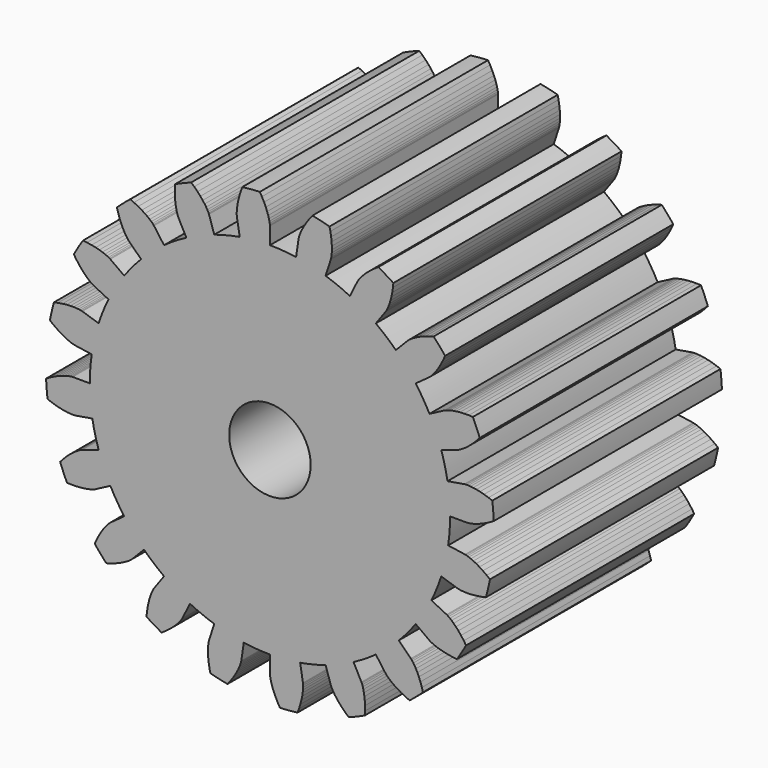
from build123d import *

# Parameters (mm, degrees)
F0_R     = 5
F1_DEPTH = 35


# Not quite as in the source:
# - ends of sketch curves that miss each other by under 0.0002 mm in the source are joined


with BuildPart() as f1:
    # F0 (on Front) → F1 (new body)
    with BuildSketch(Plane.XZ):
        with BuildLine():
            Line((-22.108, 0), (-24.2, 0))
            Line((-24.2, 0), (-24.23024, -0.00108))
            Line((-24.23024, -0.00108), (-24.32068, -0.00824))
            Line((-24.32068, -0.00824), (-24.47072, -0.02744))
            Line((-24.47072, -0.02744), (-24.67916, -0.06464))
            Line((-24.67916, -0.06464), (-24.94448, -0.12572))
            Line((-24.94448, -0.12572), (-25.2646, -0.2164))
            Line((-25.2646, -0.2164), (-25.63716, -0.34232))
            Line((-25.63716, -0.34232), (-26.05924, -0.50884))
            Line((-26.05924, -0.50884), (-26.52756, -0.72116))
            Line((-26.52756, -0.72116), (-27.03852, -0.98436))
            Line((-27.03852, -0.98436), (-27.4722, -1.23588))
            ThreePointArc((-27.4722, -1.23588), (-27.4025906987, -2.3125792959), (-27.2907844004, -3.3857180647))
            Line((-27.2907844004, -3.3857180647), (-26.82104, -3.561))
            Line((-26.82104, -3.561), (-26.27324, -3.73484))
            Line((-26.27324, -3.73484), (-25.77592, -3.86568))
            Line((-25.77592, -3.86568), (-25.33192, -3.95912))
            Line((-25.33192, -3.95912), (-24.94356, -4.0208))
            Line((-24.94356, -4.0208), (-24.61272, -4.05656))
            Line((-24.61272, -4.05656), (-24.34096, -4.07228))
            Line((-24.34096, -4.07228), (-24.1292, -4.07404))
            Line((-24.1292, -4.07404), (-23.97808, -4.06784))
            Line((-23.97808, -4.06784), (-23.88772, -4.05972))
            Line((-23.88772, -4.05972), (-23.85772, -4.05572))
            Line((-23.85772, -4.05572), (-21.79532, -3.70512))
            ThreePointArc((-21.79532, -3.70512), (-21.4676323683, -5.2824638663), (-21.0259540931, -6.8317580807))
            Line((-21.0259540931, -6.8317580807), (-23.01556, -7.4782))
            Line((-23.01556, -7.4782), (-23.044, -7.4886))
            Line((-23.044, -7.4886), (-23.1278, -7.52336))
            Line((-23.1278, -7.52336), (-23.26456, -7.58796))
            Line((-23.26456, -7.58796), (-23.45132, -7.68776))
            Line((-23.45132, -7.68776), (-23.68476, -7.82784))
            Line((-23.68476, -7.82784), (-23.9612, -8.013))
            Line((-23.9612, -8.013), (-24.2766, -8.24788))
            Line((-24.2766, -8.24788), (-24.62656, -8.53668))
            Line((-24.62656, -8.53668), (-25.00636, -8.88336))
            Line((-25.00636, -8.88336), (-25.41096, -9.29152))
            Line((-25.41096, -9.29152), (-25.74572, -9.6648))
            ThreePointArc((-25.74572, -9.6648), (-25.3467827469, -10.6672678967), (-24.9088370823, -11.653318635))
            Line((-24.9088370823, -11.653318635), (-24.40792, -11.67488))
            Line((-24.40792, -11.67488), (-23.8332, -11.67092))
            Line((-23.8332, -11.67092), (-23.3198, -11.64168))
            Line((-23.3198, -11.64168), (-22.86864, -11.59332))
            Line((-22.86864, -11.59332), (-22.48024, -11.532))
            Line((-22.48024, -11.532), (-22.15456, -11.46376))
            Line((-22.15456, -11.46376), (-21.8912, -11.39476))
            Line((-21.8912, -11.39476), (-21.68932, -11.331))
            Line((-21.68932, -11.331), (-21.54752, -11.27836))
            Line((-21.54752, -11.27836), (-21.46404, -11.24272))
            Line((-21.46404, -11.24272), (-21.43676, -11.22964))
            Line((-21.43676, -11.22964), (-19.58364, -10.25888))
            ThreePointArc((-19.58364, -10.25888), (-18.7845703543, -11.6577691093), (-17.8857502251, -12.9947528981))
            Line((-17.8857502251, -12.9947528981), (-19.5782, -14.2244))
            Line((-19.5782, -14.2244), (-19.60204, -14.24308))
            Line((-19.60204, -14.24308), (-19.671, -14.302))
            Line((-19.671, -14.302), (-19.78112, -14.40572))
            Line((-19.78112, -14.40572), (-19.92788, -14.55836))
            Line((-19.92788, -14.55836), (-20.1066, -14.76368))
            Line((-20.1066, -14.76368), (-20.31232, -15.02524))
            Line((-20.31232, -15.02524), (-20.53968, -15.34608))
            Line((-20.53968, -15.34608), (-20.78328, -15.72888))
            Line((-20.78328, -15.72888), (-21.03736, -16.17596))
            Line((-21.03736, -16.17596), (-21.29604, -16.6892))
            Line((-21.29604, -16.6892), (-21.49904, -17.1476))
            ThreePointArc((-21.49904, -17.1476), (-20.8098683635, -17.9777467635), (-20.0886483796, -18.7802078338))
            Line((-20.0886483796, -18.7802078338), (-19.6056, -18.64592))
            Line((-19.6056, -18.64592), (-19.06024, -18.46456))
            Line((-19.06024, -18.46456), (-18.58096, -18.27812))
            Line((-18.58096, -18.27812), (-18.16684, -18.09272))
            Line((-18.16684, -18.09272), (-17.8164, -17.91436))
            Line((-17.8164, -17.91436), (-17.52776, -17.74884))
            Line((-17.52776, -17.74884), (-17.2986, -17.6018))
            Line((-17.2986, -17.6018), (-17.12628, -17.47876))
            Line((-17.12628, -17.47876), (-17.00768, -17.38492))
            Line((-17.00768, -17.38492), (-16.93932, -17.3252))
            Line((-16.93932, -17.3252), (-16.9174, -17.30436))
            Line((-16.9174, -17.30436), (-15.45496, -15.80848))
            ThreePointArc((-15.45496, -15.80848), (-14.2627230801, -16.8919624183), (-12.9947528981, -17.8857502251))
            Line((-12.9947528981, -17.8857502251), (-14.2244, -19.5782))
            Line((-14.2244, -19.5782), (-14.24128, -19.60332))
            Line((-14.24128, -19.60332), (-14.28868, -19.68068))
            Line((-14.28868, -19.68068), (-14.36132, -19.81336))
            Line((-14.36132, -19.81336), (-14.45376, -20.00388))
            Line((-14.45376, -20.00388), (-14.56028, -20.2544))
            Line((-14.56028, -20.2544), (-14.67508, -20.56672))
            Line((-14.67508, -20.56672), (-14.7922, -20.94208))
            Line((-14.7922, -20.94208), (-14.9056, -21.38144))
            Line((-14.9056, -21.38144), (-15.00908, -21.88516))
            Line((-15.00908, -21.88516), (-15.09648, -22.4532))
            Line((-15.09648, -22.4532), (-15.14792, -22.95192))
            ThreePointArc((-15.14792, -22.95192), (-14.2359384688, -23.5284520509), (-13.3020446076, -24.068768337))
            Line((-13.3020446076, -24.068768337), (-12.88412, -23.7918))
            Line((-12.88412, -23.7918), (-12.42148, -23.45076))
            Line((-12.42148, -23.45076), (-12.02332, -23.12536))
            Line((-12.02332, -23.12536), (-11.68676, -22.82108))
            Line((-11.68676, -22.82108), (-11.40856, -22.54312))
            Line((-11.40856, -22.54312), (-11.1852, -22.29652))
            Line((-11.1852, -22.29652), (-11.01268, -22.08588))
            Line((-11.01268, -22.08588), (-10.88684, -21.9156))
            Line((-10.88684, -21.9156), (-10.80304, -21.78968))
            Line((-10.80304, -21.78968), (-10.75648, -21.7118))
            Line((-10.75648, -21.7118), (-10.74208, -21.6852))
            Line((-10.74208, -21.6852), (-9.81348, -19.8106))
            ThreePointArc((-9.81348, -19.8106), (-8.3447718051, -20.472626786), (-6.8317580807, -21.0259540931))
            Line((-6.8317580807, -21.0259540931), (-7.4782, -23.01556))
            Line((-7.4782, -23.01556), (-7.48652, -23.04464))
            Line((-7.48652, -23.04464), (-7.50768, -23.13292))
            Line((-7.50768, -23.13292), (-7.53576, -23.28152))
            Line((-7.53576, -23.28152), (-7.5648, -23.49124))
            Line((-7.5648, -23.49124), (-7.58872, -23.76244))
            Line((-7.58872, -23.76244), (-7.6014, -24.09496))
            Line((-7.6014, -24.09496), (-7.59676, -24.48816))
            Line((-7.59676, -24.48816), (-7.56884, -24.94104))
            Line((-7.56884, -24.94104), (-7.5116, -25.45208))
            Line((-7.5116, -25.45208), (-7.4192, -26.01932))
            Line((-7.4192, -26.01932), (-7.314, -26.50952))
            ThreePointArc((-7.314, -26.50952), (-6.2684865248, -26.7760354924), (-5.2133200442, -27.0013202291))
            Line((-5.2133200442, -27.0013202291), (-4.90144, -26.60876))
            Line((-4.90144, -26.60876), (-4.56684, -26.14148))
            Line((-4.56684, -26.14148), (-4.28872, -25.70892))
            Line((-4.28872, -25.70892), (-4.06264, -25.31552))
            Line((-4.06264, -25.31552), (-3.88396, -24.96524))
            Line((-3.88396, -24.96524), (-3.74776, -24.66164))
            Line((-3.74776, -24.66164), (-3.6488, -24.40804))
            Line((-3.6488, -24.40804), (-3.58168, -24.2072))
            Line((-3.58168, -24.2072), (-3.54092, -24.06156))
            Line((-3.54092, -24.06156), (-3.52072, -23.97308))
            Line((-3.52072, -23.97308), (-3.51524, -23.94332))
            Line((-3.51524, -23.94332), (-3.21136, -21.87352))
            ThreePointArc((-3.21136, -21.87352), (-1.6099544582, -22.0493018176), (0, -22.108))
            Line((0, -22.108), (0, -24.2))
            Line((0, -24.2), (0.00108, -24.23024))
            Line((0.00108, -24.23024), (0.00824, -24.32068))
            Line((0.00824, -24.32068), (0.02744, -24.47072))
            Line((0.02744, -24.47072), (0.06464, -24.67916))
            Line((0.06464, -24.67916), (0.12572, -24.94448))
            Line((0.12572, -24.94448), (0.2164, -25.2646))
            Line((0.2164, -25.2646), (0.34232, -25.63716))
            Line((0.34232, -25.63716), (0.50884, -26.05924))
            Line((0.50884, -26.05924), (0.72116, -26.52756))
            Line((0.72116, -26.52756), (0.98436, -27.03852))
            Line((0.98436, -27.03852), (1.23588, -27.4722))
            ThreePointArc((1.23588, -27.4722), (2.3125792959, -27.4025906987), (3.3857180647, -27.2907844004))
            Line((3.3857180647, -27.2907844004), (3.561, -26.82104))
            Line((3.561, -26.82104), (3.73484, -26.27324))
            Line((3.73484, -26.27324), (3.86568, -25.77592))
            Line((3.86568, -25.77592), (3.95912, -25.33192))
            Line((3.95912, -25.33192), (4.0208, -24.94356))
            Line((4.0208, -24.94356), (4.05656, -24.61272))
            Line((4.05656, -24.61272), (4.07228, -24.34096))
            Line((4.07228, -24.34096), (4.07404, -24.1292))
            Line((4.07404, -24.1292), (4.06784, -23.97808))
            Line((4.06784, -23.97808), (4.05972, -23.88772))
            Line((4.05972, -23.88772), (4.05572, -23.85772))
            Line((4.05572, -23.85772), (3.70512, -21.79532))
            ThreePointArc((3.70512, -21.79532), (5.2824638663, -21.4676323683), (6.8317580807, -21.0259540931))
            Line((6.8317580807, -21.0259540931), (7.4782, -23.01556))
            Line((7.4782, -23.01556), (7.4886, -23.044))
            Line((7.4886, -23.044), (7.52336, -23.1278))
            Line((7.52336, -23.1278), (7.58796, -23.26456))
            Line((7.58796, -23.26456), (7.68776, -23.45132))
            Line((7.68776, -23.45132), (7.82784, -23.68476))
            Line((7.82784, -23.68476), (8.013, -23.9612))
            Line((8.013, -23.9612), (8.24788, -24.2766))
            Line((8.24788, -24.2766), (8.53668, -24.62656))
            Line((8.53668, -24.62656), (8.88336, -25.00636))
            Line((8.88336, -25.00636), (9.29152, -25.41096))
            Line((9.29152, -25.41096), (9.6648, -25.74572))
            ThreePointArc((9.6648, -25.74572), (10.6672678967, -25.3467827469), (11.653318635, -24.9088370823))
            Line((11.653318635, -24.9088370823), (11.67488, -24.40792))
            Line((11.67488, -24.40792), (11.67092, -23.8332))
            Line((11.67092, -23.8332), (11.64168, -23.3198))
            Line((11.64168, -23.3198), (11.59332, -22.86864))
            Line((11.59332, -22.86864), (11.532, -22.48024))
            Line((11.532, -22.48024), (11.46376, -22.15456))
            Line((11.46376, -22.15456), (11.39476, -21.8912))
            Line((11.39476, -21.8912), (11.331, -21.68932))
            Line((11.331, -21.68932), (11.27836, -21.54752))
            Line((11.27836, -21.54752), (11.24272, -21.46404))
            Line((11.24272, -21.46404), (11.22964, -21.43676))
            Line((11.22964, -21.43676), (10.25888, -19.58364))
            ThreePointArc((10.25888, -19.58364), (11.6577691093, -18.7845703543), (12.9947528981, -17.8857502251))
            Line((12.9947528981, -17.8857502251), (14.2244, -19.5782))
            Line((14.2244, -19.5782), (14.24308, -19.60204))
            Line((14.24308, -19.60204), (14.302, -19.671))
            Line((14.302, -19.671), (14.40572, -19.78112))
            Line((14.40572, -19.78112), (14.55836, -19.92788))
            Line((14.55836, -19.92788), (14.76368, -20.1066))
            Line((14.76368, -20.1066), (15.02524, -20.31232))
            Line((15.02524, -20.31232), (15.34608, -20.53968))
            Line((15.34608, -20.53968), (15.72888, -20.78328))
            Line((15.72888, -20.78328), (16.17596, -21.03736))
            Line((16.17596, -21.03736), (16.6892, -21.29604))
            Line((16.6892, -21.29604), (17.1476, -21.49904))
            ThreePointArc((17.1476, -21.49904), (17.9777467635, -20.8098683635), (18.7802078338, -20.0886483796))
            Line((18.7802078338, -20.0886483796), (18.64592, -19.6056))
            Line((18.64592, -19.6056), (18.46456, -19.06024))
            Line((18.46456, -19.06024), (18.27812, -18.58096))
            Line((18.27812, -18.58096), (18.09272, -18.16684))
            Line((18.09272, -18.16684), (17.91436, -17.8164))
            Line((17.91436, -17.8164), (17.74884, -17.52776))
            Line((17.74884, -17.52776), (17.6018, -17.2986))
            Line((17.6018, -17.2986), (17.47876, -17.12628))
            Line((17.47876, -17.12628), (17.38492, -17.00768))
            Line((17.38492, -17.00768), (17.3252, -16.93932))
            Line((17.3252, -16.93932), (17.30436, -16.9174))
            Line((17.30436, -16.9174), (15.80848, -15.45496))
            ThreePointArc((15.80848, -15.45496), (16.8919624183, -14.2627230801), (17.8857502251, -12.9947528981))
            Line((17.8857502251, -12.9947528981), (19.5782, -14.2244))
            Line((19.5782, -14.2244), (19.60332, -14.24128))
            Line((19.60332, -14.24128), (19.68068, -14.28868))
            Line((19.68068, -14.28868), (19.81336, -14.36132))
            Line((19.81336, -14.36132), (20.00388, -14.45376))
            Line((20.00388, -14.45376), (20.2544, -14.56028))
            Line((20.2544, -14.56028), (20.56672, -14.67508))
            Line((20.56672, -14.67508), (20.94208, -14.7922))
            Line((20.94208, -14.7922), (21.38144, -14.9056))
            Line((21.38144, -14.9056), (21.88516, -15.00908))
            Line((21.88516, -15.00908), (22.4532, -15.09648))
            Line((22.4532, -15.09648), (22.95192, -15.14792))
            ThreePointArc((22.95192, -15.14792), (23.5284520509, -14.2359384688), (24.068768337, -13.3020446076))
            Line((24.068768337, -13.3020446076), (23.7918, -12.88412))
            Line((23.7918, -12.88412), (23.45076, -12.42148))
            Line((23.45076, -12.42148), (23.12536, -12.02332))
            Line((23.12536, -12.02332), (22.82108, -11.68676))
            Line((22.82108, -11.68676), (22.54312, -11.40856))
            Line((22.54312, -11.40856), (22.29652, -11.1852))
            Line((22.29652, -11.1852), (22.08588, -11.01268))
            Line((22.08588, -11.01268), (21.9156, -10.88684))
            Line((21.9156, -10.88684), (21.78968, -10.80304))
            Line((21.78968, -10.80304), (21.7118, -10.75648))
            Line((21.7118, -10.75648), (21.6852, -10.74208))
            Line((21.6852, -10.74208), (19.8106, -9.81348))
            ThreePointArc((19.8106, -9.81348), (20.472626786, -8.3447718051), (21.0259540931, -6.8317580807))
            Line((21.0259540931, -6.8317580807), (23.01556, -7.4782))
            Line((23.01556, -7.4782), (23.04464, -7.48652))
            Line((23.04464, -7.48652), (23.13292, -7.50768))
            Line((23.13292, -7.50768), (23.28152, -7.53576))
            Line((23.28152, -7.53576), (23.49124, -7.5648))
            Line((23.49124, -7.5648), (23.76244, -7.58872))
            Line((23.76244, -7.58872), (24.09496, -7.6014))
            Line((24.09496, -7.6014), (24.48816, -7.59676))
            Line((24.48816, -7.59676), (24.94104, -7.56884))
            Line((24.94104, -7.56884), (25.45208, -7.5116))
            Line((25.45208, -7.5116), (26.01932, -7.4192))
            Line((26.01932, -7.4192), (26.50952, -7.314))
            ThreePointArc((26.50952, -7.314), (26.7760354924, -6.2684865248), (27.0013202291, -5.2133200442))
            Line((27.0013202291, -5.2133200442), (26.60876, -4.90144))
            Line((26.60876, -4.90144), (26.14148, -4.56684))
            Line((26.14148, -4.56684), (25.70892, -4.28872))
            Line((25.70892, -4.28872), (25.31552, -4.06264))
            Line((25.31552, -4.06264), (24.96524, -3.88396))
            Line((24.96524, -3.88396), (24.66164, -3.74776))
            Line((24.66164, -3.74776), (24.40804, -3.6488))
            Line((24.40804, -3.6488), (24.2072, -3.58168))
            Line((24.2072, -3.58168), (24.06156, -3.54092))
            Line((24.06156, -3.54092), (23.97308, -3.52072))
            Line((23.97308, -3.52072), (23.94332, -3.51524))
            Line((23.94332, -3.51524), (21.87352, -3.21136))
            ThreePointArc((21.87352, -3.21136), (22.0493018176, -1.6099544582), (22.108, 0))
            Line((22.108, 0), (24.2, 0))
            Line((24.2, 0), (24.23024, 0.00108))
            Line((24.23024, 0.00108), (24.32068, 0.00824))
            Line((24.32068, 0.00824), (24.47072, 0.02744))
            Line((24.47072, 0.02744), (24.67916, 0.06464))
            Line((24.67916, 0.06464), (24.94448, 0.12572))
            Line((24.94448, 0.12572), (25.2646, 0.2164))
            Line((25.2646, 0.2164), (25.63716, 0.34232))
            Line((25.63716, 0.34232), (26.05924, 0.50884))
            Line((26.05924, 0.50884), (26.52756, 0.72116))
            Line((26.52756, 0.72116), (27.03852, 0.98436))
            Line((27.03852, 0.98436), (27.4722, 1.23588))
            ThreePointArc((27.4722, 1.23588), (27.4025906987, 2.3125792959), (27.2907844004, 3.3857180647))
            Line((27.2907844004, 3.3857180647), (26.82104, 3.561))
            Line((26.82104, 3.561), (26.27324, 3.73484))
            Line((26.27324, 3.73484), (25.77592, 3.86568))
            Line((25.77592, 3.86568), (25.33192, 3.95912))
            Line((25.33192, 3.95912), (24.94356, 4.0208))
            Line((24.94356, 4.0208), (24.61272, 4.05656))
            Line((24.61272, 4.05656), (24.34096, 4.07228))
            Line((24.34096, 4.07228), (24.1292, 4.07404))
            Line((24.1292, 4.07404), (23.97808, 4.06784))
            Line((23.97808, 4.06784), (23.88772, 4.05972))
            Line((23.88772, 4.05972), (23.85772, 4.05572))
            Line((23.85772, 4.05572), (21.79532, 3.70512))
            ThreePointArc((21.79532, 3.70512), (21.4676323683, 5.2824638663), (21.0259540931, 6.8317580807))
            Line((21.0259540931, 6.8317580807), (23.01556, 7.4782))
            Line((23.01556, 7.4782), (23.044, 7.4886))
            Line((23.044, 7.4886), (23.1278, 7.52336))
            Line((23.1278, 7.52336), (23.26456, 7.58796))
            Line((23.26456, 7.58796), (23.45132, 7.68776))
            Line((23.45132, 7.68776), (23.68476, 7.82784))
            Line((23.68476, 7.82784), (23.9612, 8.013))
            Line((23.9612, 8.013), (24.2766, 8.24788))
            Line((24.2766, 8.24788), (24.62656, 8.53668))
            Line((24.62656, 8.53668), (25.00636, 8.88336))
            Line((25.00636, 8.88336), (25.41096, 9.29152))
            Line((25.41096, 9.29152), (25.74572, 9.6648))
            ThreePointArc((25.74572, 9.6648), (25.3467827469, 10.6672678967), (24.9088370823, 11.653318635))
            Line((24.9088370823, 11.653318635), (24.40792, 11.67488))
            Line((24.40792, 11.67488), (23.8332, 11.67092))
            Line((23.8332, 11.67092), (23.3198, 11.64168))
            Line((23.3198, 11.64168), (22.86864, 11.59332))
            Line((22.86864, 11.59332), (22.48024, 11.532))
            Line((22.48024, 11.532), (22.15456, 11.46376))
            Line((22.15456, 11.46376), (21.8912, 11.39476))
            Line((21.8912, 11.39476), (21.68932, 11.331))
            Line((21.68932, 11.331), (21.54752, 11.27836))
            Line((21.54752, 11.27836), (21.46404, 11.24272))
            Line((21.46404, 11.24272), (21.43676, 11.22964))
            Line((21.43676, 11.22964), (19.58364, 10.25888))
            ThreePointArc((19.58364, 10.25888), (18.7845703543, 11.6577691093), (17.8857502251, 12.9947528981))
            Line((17.8857502251, 12.9947528981), (19.5782, 14.2244))
            Line((19.5782, 14.2244), (19.60204, 14.24308))
            Line((19.60204, 14.24308), (19.671, 14.302))
            Line((19.671, 14.302), (19.78112, 14.40572))
            Line((19.78112, 14.40572), (19.92788, 14.55836))
            Line((19.92788, 14.55836), (20.1066, 14.76368))
            Line((20.1066, 14.76368), (20.31232, 15.02524))
            Line((20.31232, 15.02524), (20.53968, 15.34608))
            Line((20.53968, 15.34608), (20.78328, 15.72888))
            Line((20.78328, 15.72888), (21.03736, 16.17596))
            Line((21.03736, 16.17596), (21.29604, 16.6892))
            Line((21.29604, 16.6892), (21.49904, 17.1476))
            ThreePointArc((21.49904, 17.1476), (20.8098683635, 17.9777467635), (20.0886483796, 18.7802078338))
            Line((20.0886483796, 18.7802078338), (19.6056, 18.64592))
            Line((19.6056, 18.64592), (19.06024, 18.46456))
            Line((19.06024, 18.46456), (18.58096, 18.27812))
            Line((18.58096, 18.27812), (18.16684, 18.09272))
            Line((18.16684, 18.09272), (17.8164, 17.91436))
            Line((17.8164, 17.91436), (17.52776, 17.74884))
            Line((17.52776, 17.74884), (17.2986, 17.6018))
            Line((17.2986, 17.6018), (17.12628, 17.47876))
            Line((17.12628, 17.47876), (17.00768, 17.38492))
            Line((17.00768, 17.38492), (16.93932, 17.3252))
            Line((16.93932, 17.3252), (16.9174, 17.30436))
            Line((16.9174, 17.30436), (15.45496, 15.80848))
            ThreePointArc((15.45496, 15.80848), (14.2627230801, 16.8919624183), (12.9947528981, 17.8857502251))
            Line((12.9947528981, 17.8857502251), (14.2244, 19.5782))
            Line((14.2244, 19.5782), (14.24128, 19.60332))
            Line((14.24128, 19.60332), (14.28868, 19.68068))
            Line((14.28868, 19.68068), (14.36132, 19.81336))
            Line((14.36132, 19.81336), (14.45376, 20.00388))
            Line((14.45376, 20.00388), (14.56028, 20.2544))
            Line((14.56028, 20.2544), (14.67508, 20.56672))
            Line((14.67508, 20.56672), (14.7922, 20.94208))
            Line((14.7922, 20.94208), (14.9056, 21.38144))
            Line((14.9056, 21.38144), (15.00908, 21.88516))
            Line((15.00908, 21.88516), (15.09648, 22.4532))
            Line((15.09648, 22.4532), (15.14792, 22.95192))
            ThreePointArc((15.14792, 22.95192), (14.2359384688, 23.5284520509), (13.3020446076, 24.068768337))
            Line((13.3020446076, 24.068768337), (12.88412, 23.7918))
            Line((12.88412, 23.7918), (12.42148, 23.45076))
            Line((12.42148, 23.45076), (12.02332, 23.12536))
            Line((12.02332, 23.12536), (11.68676, 22.82108))
            Line((11.68676, 22.82108), (11.40856, 22.54312))
            Line((11.40856, 22.54312), (11.1852, 22.29652))
            Line((11.1852, 22.29652), (11.01268, 22.08588))
            Line((11.01268, 22.08588), (10.88684, 21.9156))
            Line((10.88684, 21.9156), (10.80304, 21.78968))
            Line((10.80304, 21.78968), (10.75648, 21.7118))
            Line((10.75648, 21.7118), (10.74208, 21.6852))
            Line((10.74208, 21.6852), (9.81348, 19.8106))
            ThreePointArc((9.81348, 19.8106), (8.3447718051, 20.472626786), (6.8317580807, 21.0259540931))
            Line((6.8317580807, 21.0259540931), (7.4782, 23.01556))
            Line((7.4782, 23.01556), (7.48652, 23.04464))
            Line((7.48652, 23.04464), (7.50768, 23.13292))
            Line((7.50768, 23.13292), (7.53576, 23.28152))
            Line((7.53576, 23.28152), (7.5648, 23.49124))
            Line((7.5648, 23.49124), (7.58872, 23.76244))
            Line((7.58872, 23.76244), (7.6014, 24.09496))
            Line((7.6014, 24.09496), (7.59676, 24.48816))
            Line((7.59676, 24.48816), (7.56884, 24.94104))
            Line((7.56884, 24.94104), (7.5116, 25.45208))
            Line((7.5116, 25.45208), (7.4192, 26.01932))
            Line((7.4192, 26.01932), (7.314, 26.50952))
            ThreePointArc((7.314, 26.50952), (6.2684865248, 26.7760354924), (5.2133200442, 27.0013202291))
            Line((5.2133200442, 27.0013202291), (4.90144, 26.60876))
            Line((4.90144, 26.60876), (4.56684, 26.14148))
            Line((4.56684, 26.14148), (4.28872, 25.70892))
            Line((4.28872, 25.70892), (4.06264, 25.31552))
            Line((4.06264, 25.31552), (3.88396, 24.96524))
            Line((3.88396, 24.96524), (3.74776, 24.66164))
            Line((3.74776, 24.66164), (3.6488, 24.40804))
            Line((3.6488, 24.40804), (3.58168, 24.2072))
            Line((3.58168, 24.2072), (3.54092, 24.06156))
            Line((3.54092, 24.06156), (3.52072, 23.97308))
            Line((3.52072, 23.97308), (3.51524, 23.94332))
            Line((3.51524, 23.94332), (3.21136, 21.87352))
            ThreePointArc((3.21136, 21.87352), (1.6099544582, 22.0493018176), (0, 22.108))
            Line((0, 22.108), (0, 24.2))
            Line((0, 24.2), (-0.00108, 24.23024))
            Line((-0.00108, 24.23024), (-0.00824, 24.32068))
            Line((-0.00824, 24.32068), (-0.02744, 24.47072))
            Line((-0.02744, 24.47072), (-0.06464, 24.67916))
            Line((-0.06464, 24.67916), (-0.12572, 24.94448))
            Line((-0.12572, 24.94448), (-0.2164, 25.2646))
            Line((-0.2164, 25.2646), (-0.34232, 25.63716))
            Line((-0.34232, 25.63716), (-0.50884, 26.05924))
            Line((-0.50884, 26.05924), (-0.72116, 26.52756))
            Line((-0.72116, 26.52756), (-0.98436, 27.03852))
            Line((-0.98436, 27.03852), (-1.23588, 27.4722))
            ThreePointArc((-1.23588, 27.4722), (-2.3125792959, 27.4025906987), (-3.3857180647, 27.2907844004))
            Line((-3.3857180647, 27.2907844004), (-3.561, 26.82104))
            Line((-3.561, 26.82104), (-3.73484, 26.27324))
            Line((-3.73484, 26.27324), (-3.86568, 25.77592))
            Line((-3.86568, 25.77592), (-3.95912, 25.33192))
            Line((-3.95912, 25.33192), (-4.0208, 24.94356))
            Line((-4.0208, 24.94356), (-4.05656, 24.61272))
            Line((-4.05656, 24.61272), (-4.07228, 24.34096))
            Line((-4.07228, 24.34096), (-4.07404, 24.1292))
            Line((-4.07404, 24.1292), (-4.06784, 23.97808))
            Line((-4.06784, 23.97808), (-4.05972, 23.88772))
            Line((-4.05972, 23.88772), (-4.05572, 23.85772))
            Line((-4.05572, 23.85772), (-3.70512, 21.79532))
            ThreePointArc((-3.70512, 21.79532), (-5.2824638663, 21.4676323683), (-6.8317580807, 21.0259540931))
            Line((-6.8317580807, 21.0259540931), (-7.4782, 23.01556))
            Line((-7.4782, 23.01556), (-7.4886, 23.044))
            Line((-7.4886, 23.044), (-7.52336, 23.1278))
            Line((-7.52336, 23.1278), (-7.58796, 23.26456))
            Line((-7.58796, 23.26456), (-7.68776, 23.45132))
            Line((-7.68776, 23.45132), (-7.82784, 23.68476))
            Line((-7.82784, 23.68476), (-8.013, 23.9612))
            Line((-8.013, 23.9612), (-8.24788, 24.2766))
            Line((-8.24788, 24.2766), (-8.53668, 24.62656))
            Line((-8.53668, 24.62656), (-8.88336, 25.00636))
            Line((-8.88336, 25.00636), (-9.29152, 25.41096))
            Line((-9.29152, 25.41096), (-9.6648, 25.74572))
            ThreePointArc((-9.6648, 25.74572), (-10.6672678967, 25.3467827469), (-11.653318635, 24.9088370823))
            Line((-11.653318635, 24.9088370823), (-11.67488, 24.40792))
            Line((-11.67488, 24.40792), (-11.67092, 23.8332))
            Line((-11.67092, 23.8332), (-11.64168, 23.3198))
            Line((-11.64168, 23.3198), (-11.59332, 22.86864))
            Line((-11.59332, 22.86864), (-11.532, 22.48024))
            Line((-11.532, 22.48024), (-11.46376, 22.15456))
            Line((-11.46376, 22.15456), (-11.39476, 21.8912))
            Line((-11.39476, 21.8912), (-11.331, 21.68932))
            Line((-11.331, 21.68932), (-11.27836, 21.54752))
            Line((-11.27836, 21.54752), (-11.24272, 21.46404))
            Line((-11.24272, 21.46404), (-11.22964, 21.43676))
            Line((-11.22964, 21.43676), (-10.25888, 19.58364))
            ThreePointArc((-10.25888, 19.58364), (-11.6577691093, 18.7845703543), (-12.9947528981, 17.8857502251))
            Line((-12.9947528981, 17.8857502251), (-14.2244, 19.5782))
            Line((-14.2244, 19.5782), (-14.24308, 19.60204))
            Line((-14.24308, 19.60204), (-14.302, 19.671))
            Line((-14.302, 19.671), (-14.40572, 19.78112))
            Line((-14.40572, 19.78112), (-14.55836, 19.92788))
            Line((-14.55836, 19.92788), (-14.76368, 20.1066))
            Line((-14.76368, 20.1066), (-15.02524, 20.31232))
            Line((-15.02524, 20.31232), (-15.34608, 20.53968))
            Line((-15.34608, 20.53968), (-15.72888, 20.78328))
            Line((-15.72888, 20.78328), (-16.17596, 21.03736))
            Line((-16.17596, 21.03736), (-16.6892, 21.29604))
            Line((-16.6892, 21.29604), (-17.1476, 21.49904))
            ThreePointArc((-17.1476, 21.49904), (-17.9777467635, 20.8098683635), (-18.7802078338, 20.0886483796))
            Line((-18.7802078338, 20.0886483796), (-18.64592, 19.6056))
            Line((-18.64592, 19.6056), (-18.46456, 19.06024))
            Line((-18.46456, 19.06024), (-18.27812, 18.58096))
            Line((-18.27812, 18.58096), (-18.09272, 18.16684))
            Line((-18.09272, 18.16684), (-17.91436, 17.8164))
            Line((-17.91436, 17.8164), (-17.74884, 17.52776))
            Line((-17.74884, 17.52776), (-17.6018, 17.2986))
            Line((-17.6018, 17.2986), (-17.47876, 17.12628))
            Line((-17.47876, 17.12628), (-17.38492, 17.00768))
            Line((-17.38492, 17.00768), (-17.3252, 16.93932))
            Line((-17.3252, 16.93932), (-17.30436, 16.9174))
            Line((-17.30436, 16.9174), (-15.80848, 15.45496))
            ThreePointArc((-15.80848, 15.45496), (-16.8919624183, 14.2627230801), (-17.8857502251, 12.9947528981))
            Line((-17.8857502251, 12.9947528981), (-19.5782, 14.2244))
            Line((-19.5782, 14.2244), (-19.60332, 14.24128))
            Line((-19.60332, 14.24128), (-19.68068, 14.28868))
            Line((-19.68068, 14.28868), (-19.81336, 14.36132))
            Line((-19.81336, 14.36132), (-20.00388, 14.45376))
            Line((-20.00388, 14.45376), (-20.2544, 14.56028))
            Line((-20.2544, 14.56028), (-20.56672, 14.67508))
            Line((-20.56672, 14.67508), (-20.94208, 14.7922))
            Line((-20.94208, 14.7922), (-21.38144, 14.9056))
            Line((-21.38144, 14.9056), (-21.88516, 15.00908))
            Line((-21.88516, 15.00908), (-22.4532, 15.09648))
            Line((-22.4532, 15.09648), (-22.95192, 15.14792))
            ThreePointArc((-22.95192, 15.14792), (-23.5284520509, 14.2359384688), (-24.068768337, 13.3020446076))
            Line((-24.068768337, 13.3020446076), (-23.7918, 12.88412))
            Line((-23.7918, 12.88412), (-23.45076, 12.42148))
            Line((-23.45076, 12.42148), (-23.12536, 12.02332))
            Line((-23.12536, 12.02332), (-22.82108, 11.68676))
            Line((-22.82108, 11.68676), (-22.54312, 11.40856))
            Line((-22.54312, 11.40856), (-22.29652, 11.1852))
            Line((-22.29652, 11.1852), (-22.08588, 11.01268))
            Line((-22.08588, 11.01268), (-21.9156, 10.88684))
            Line((-21.9156, 10.88684), (-21.78968, 10.80304))
            Line((-21.78968, 10.80304), (-21.7118, 10.75648))
            Line((-21.7118, 10.75648), (-21.6852, 10.74208))
            Line((-21.6852, 10.74208), (-19.8106, 9.81348))
            ThreePointArc((-19.8106, 9.81348), (-20.472626786, 8.3447718051), (-21.0259540931, 6.8317580807))
            Line((-21.0259540931, 6.8317580807), (-23.01556, 7.4782))
            Line((-23.01556, 7.4782), (-23.04464, 7.48652))
            Line((-23.04464, 7.48652), (-23.13292, 7.50768))
            Line((-23.13292, 7.50768), (-23.28152, 7.53576))
            Line((-23.28152, 7.53576), (-23.49124, 7.5648))
            Line((-23.49124, 7.5648), (-23.76244, 7.58872))
            Line((-23.76244, 7.58872), (-24.09496, 7.6014))
            Line((-24.09496, 7.6014), (-24.48816, 7.59676))
            Line((-24.48816, 7.59676), (-24.94104, 7.56884))
            Line((-24.94104, 7.56884), (-25.45208, 7.5116))
            Line((-25.45208, 7.5116), (-26.01932, 7.4192))
            Line((-26.01932, 7.4192), (-26.50952, 7.314))
            ThreePointArc((-26.50952, 7.314), (-26.7760354924, 6.2684865248), (-27.0013202291, 5.2133200442))
            Line((-27.0013202291, 5.2133200442), (-26.60876, 4.90144))
            Line((-26.60876, 4.90144), (-26.14148, 4.56684))
            Line((-26.14148, 4.56684), (-25.70892, 4.28872))
            Line((-25.70892, 4.28872), (-25.31552, 4.06264))
            Line((-25.31552, 4.06264), (-24.96524, 3.88396))
            Line((-24.96524, 3.88396), (-24.66164, 3.74776))
            Line((-24.66164, 3.74776), (-24.40804, 3.6488))
            Line((-24.40804, 3.6488), (-24.2072, 3.58168))
            Line((-24.2072, 3.58168), (-24.06156, 3.54092))
            Line((-24.06156, 3.54092), (-23.97308, 3.52072))
            Line((-23.97308, 3.52072), (-23.94332, 3.51524))
            Line((-23.94332, 3.51524), (-21.87352, 3.21136))
            ThreePointArc((-21.87352, 3.21136), (-22.0493018176, 1.6099544582), (-22.108, 0))
        make_face()
        Circle(F0_R, mode=Mode.SUBTRACT)
    extrude(amount=F1_DEPTH)


solid = f1.part
